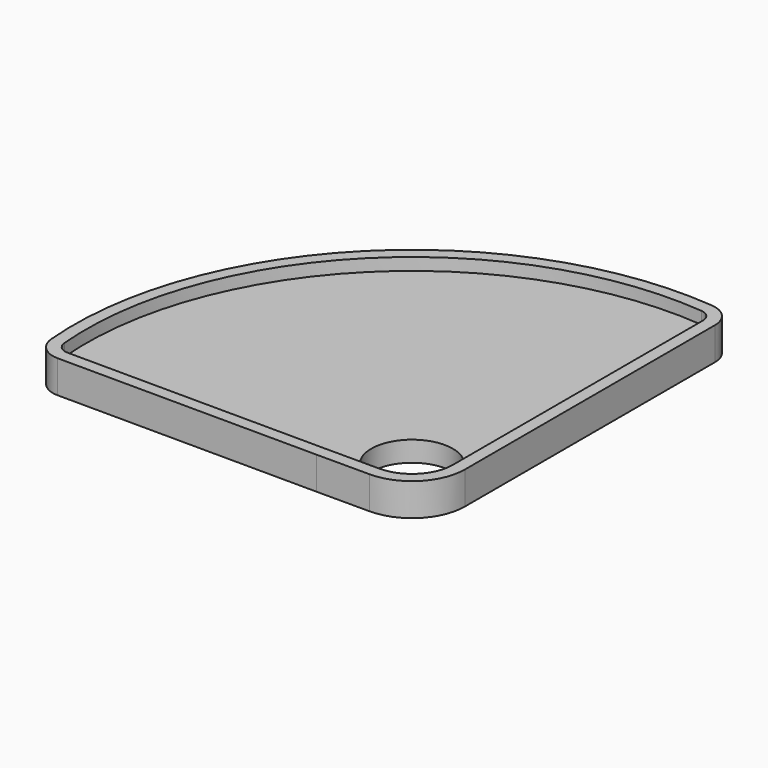
from build123d import *

# Parameters (mm, degrees)
F1_DEPTH = 4
F2_T     = -1.5
F5_DEPTH = 2.5
F7_DEPTH = 4.001
F8_R     = 3
F9_R     = 1.5


# Not quite as in the source:
# - a feature names something its author has since deleted; it is built from what else it names


with BuildPart() as f1:
    # F0 (on Top) → F1 (new body)
    with BuildSketch(Plane.XY):
        with BuildLine():
            ThreePointArc((-6.5, 0), (-1.9038059223, 1.9038059223), (0, 6.5))
            Line((0, 6.5), (0, 47.4878030638))
            ThreePointArc((0, 47.4878030638), (-35.79631442, 35.8934680057), (-47.5090982427, 0.1357356025))
            Line((-47.5090982427, 0.1357356025), (-13, 0))
            Line((-13, 0), (-6.5, 0))
        make_face()
    extrude(amount=F1_DEPTH)

    # F2
    f2_openings = [f1.faces().sort_by_distance(p)[0] for p in [
        (-21.256566, 21.300379, 4),
        (-21.256566, 21.300379, 0),
    ]]
    offset(amount=F2_T, openings=f2_openings)

    # F4 (on offset) → F5 (join)
    with BuildSketch(Plane.XY.offset(2.5)):
        with BuildLine():
            Line((-46.2025064836, 1.6306079518), (-12.9970500154, 1.5))
            Line((-12.9970500154, 1.5), (-6.5, 1.5))
            ThreePointArc((-6.5, 1.5), (-2.9644660941, 2.9644660941), (-1.5, 6.5))
            Line((-1.5, 6.5), (-1.5, 46.186269666))
            ThreePointArc((-1.5, 46.186269666), (-34.737700628, 34.8307653134), (-46.2025064836, 1.6306079518))
        make_face()
    extrude(amount=-F5_DEPTH)

    # F6 (on face) → F7 (cut, through all)
    with BuildSketch(Plane.XY.offset(4)):
        with BuildLine():
            ThreePointArc((-1.5, 6.5), (-10.0355339059, 10.0355339059), (-6.5, 1.5))
            ThreePointArc((-6.5, 1.5), (-2.9644660941, 2.9644660941), (-1.5, 6.5))
        make_face()
    extrude(amount=-F7_DEPTH, mode=Mode.SUBTRACT)

    # F8
    f8_edges = [f1.edges().sort_by_distance(p)[0] for p in [
        (-47.509098, 0.135736, 2),
        (0, 47.487803, 2),
    ]]
    fillet(f8_edges, radius=F8_R)

    # F9
    f9_edges = [f1.edges().sort_by_distance(p)[0] for p in [
        (-46.202506, 1.630608, 3.25),
        (-1.5, 46.18627, 3.25),
    ]]
    fillet(f9_edges, radius=F9_R)


solid = f1.part
